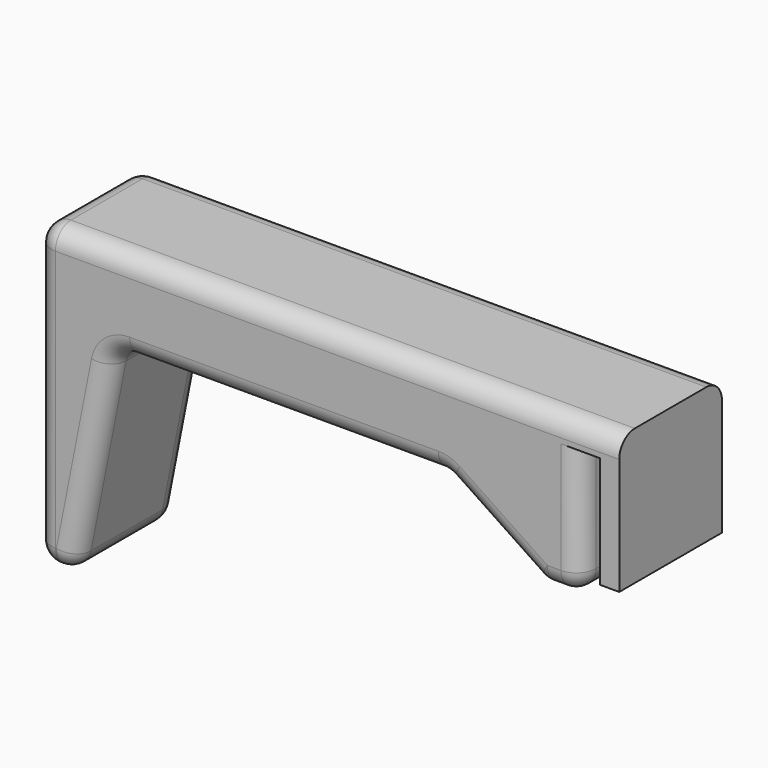
from build123d import *

# Parameters (mm, degrees)
F1_DEPTH = 33
F2_F1_R  = 5
F2_F2_R  = 5


with BuildPart() as f1:
    # F0 (on Front) → F1 (new body)
    with BuildSketch(Plane.XZ):
        Polygon((44.3557138985, 43.3492468083), (-95.6442861015, 43.3492468083), (-95.6442861015, -33.8743397176), (-86.2685606181, -33.8743397176), (-75.6651710416, 20.0938743485), (9.3348289584, 20.0938743485), (34.3557138985, 3.3492468083), (44.3557138985, 3.3492468083), (44.3557138985, 37.0205976069), align=None)
        Polygon((54.3557138985, 43.3492468083), (44.3557138985, 43.3492468083), (44.3557138985, 37.0205976069), (49.4557138985, 37.0205976069), (49.4557138985, 8.3492468083), (54.3557138985, 8.3492468083), align=None)
    extrude(amount=F1_DEPTH)

    # F2: fillet of radius 5 on 19 edges, made by hand

    # F2_f1
    f2_f1_edges = [f1.edges().sort_by_distance(p)[0] for p in [
        (-75.6651710416, -16.5, 20.0938743485),
        (9.3348289584, -16.5, 20.0938743485),
    ]]
    fillet(f2_f1_edges, radius=F2_F1_R)

    # F2_f2
    f2_f2_edges = [f1.edges().sort_by_distance(p)[0] for p in [
        (-31.8679165952, 0, 20.0938743485),
        (-31.8679165952, -33, 20.0938743485),
        (-95.6442861015, -16.5, -33.8743397176),
        (-86.2685606181, -16.5, -33.8743397176),
        (-90.9564233598, 0, -33.8743397176),
        (-90.9564233598, -33, -33.8743397176),
        (-95.6442861015, -16.5, 43.3492468083),
        (-95.6442861015, 0, 4.7374535453),
        (-95.6442861015, -33, 4.7374535453),
        (-20.6442861015, 0, 43.3492468083),
        (-20.6442861015, -33, 43.3492468083),
        (34.3557138985, -16.5, 3.3492468083),
        (44.3557138985, -33, 20.1849222076),
        (44.3557138985, 0, 20.1849222076),
        (44.3557138985, -16.5, 3.3492468083),
        (39.3557138985, 0, 3.3492468083),
        (39.3557138985, -33, 3.3492468083),
        (-74.7284504953, -33, 18.9552032994),
        (9.2692742039, -33, 19.8780504751),
        (-74.7284504953, 0, 18.9552032994),
        (9.2692742039, 0, 19.8780504751),
    ]]
    fillet(f2_f2_edges, radius=F2_F2_R)


solid = f1.part
